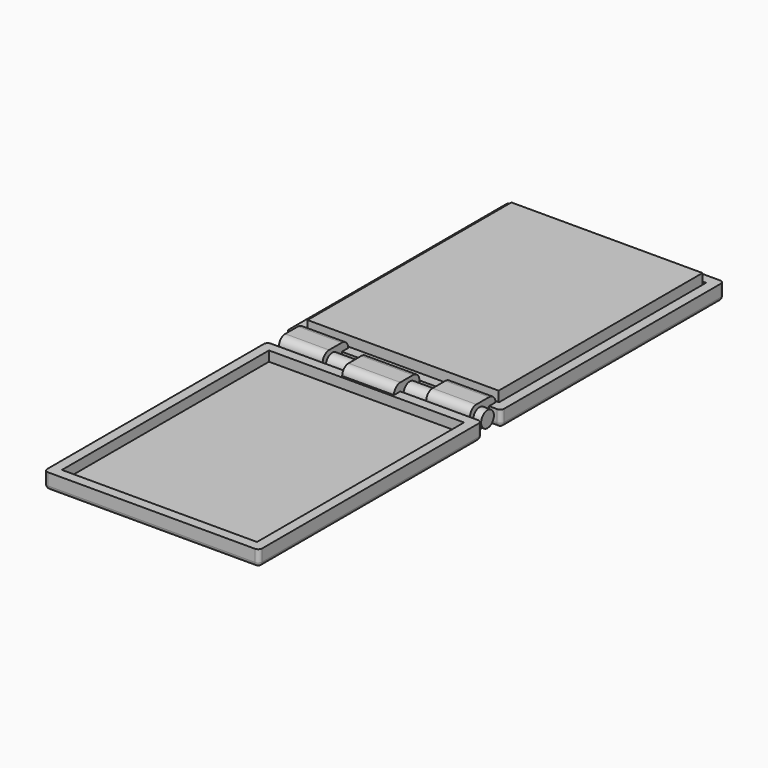
from build123d import *

# Parameters (mm, degrees)
F0_W      = 24
F0_H      = 32
F1_DEPTH  = 2.1
F3_W      = 27.0000016689
F3_H      = 35.0000016689
F3_W_2    = 24
F3_H_2    = 32
F4_DEPTH  = 4
F6_OFFSET = 0.25
F7_R      = 0.5
F5_W      = 35.0000016689
F5_H      = 2
F8_DEPTH  = 27.0000016689
F11_W     = 6.5
F11_H     = 2.9999983311
F11_H_2   = 1
F12_DEPTH = 3
F11_W_2   = 5.5000003338
F11_W_3   = 5.5000004172
F13_R     = 1
F14_DEPTH = 25
F15_R     = 1
F15_2_R   = 1
F15_3_R   = 1


with BuildPart() as f1:
    # F0 (on Top) → F1 (new body)
    with BuildSketch(Plane.XY):
        with Locations((12, 16)):
            Rectangle(F0_W, F0_H)
    extrude(amount=F1_DEPTH)


with BuildPart() as f4:
    # F3 (on offset) → F4 (new body)
    with BuildSketch(Plane.XY.offset(-1)):
        with Locations((12, 16)):
            Rectangle(F3_W, F3_H)
        with Locations((12, 16)):
            Rectangle(F3_W_2, F3_H_2, mode=Mode.SUBTRACT)
        with Locations((12, 16)):
            Rectangle(F3_W_2, F3_H_2)
    extrude(amount=F4_DEPTH)

    # F6: cut F1, made larger all round first
    f6_tool = offset(f1.part, amount=F6_OFFSET, kind=Kind.INTERSECTION, mode=Mode.PRIVATE)
    add(f6_tool, mode=Mode.SUBTRACT)

    # F7
    f7_edges = [f4.edges().sort_by_distance(p)[0] for p in [
        (-1.500001, -1.500001, 1),
        (25.500001, -1.500001, 1),
        (25.500001, 33.500001, 1),
        (-1.500001, 33.500001, 1),
        (-1.500001, 16, 3),
        (12, 33.500001, 3),
        (12, 33.500001, -1),
        (-1.500001, 16, -1),
        (25.500001, 16, 3),
        (25.500001, 16, -1),
        (12, -1.500001, 3),
        (12, -1.500001, -1),
    ]]
    fillet(f7_edges, radius=F7_R)

    # F5 (on face) → F8 (cut, through all)
    with BuildSketch(Plane.YZ.offset(25.5000008345)):
        with Locations((16, 2)):
            Rectangle(F5_W, F5_H)
    extrude(amount=-F8_DEPTH, mode=Mode.SUBTRACT)


with BuildPart() as f10_1:
    # F10: instance of F4
    add(f4.part.mirror(Plane.XZ.offset(3)))


with BuildPart() as f12:
    # F11 (on offset) → F12 (new body)
    with BuildSketch(Plane.XY.offset(-1)):
        with Locations((11.9999995828, -3)):
            Rectangle(F11_W, F11_H)
        with Locations((11.9999995828, -4.9999991655)):
            Rectangle(F11_W, F11_H_2)
    extrude(amount=F12_DEPTH)

    # F15
    f15_edges = [f12.edges().sort_by_distance(p)[0] for p in [
        (12, -5.499999, 2),
        (12, -1.500001, 2),
    ]]
    fillet(f15_edges, radius=F15_R)


with BuildPart() as f12b:
    # F11 (on offset) → F12, piece 2 (new body)
    with BuildSketch(Plane.XY.offset(-1)):
        with Locations((21.2500005841, -3)):
            Rectangle(F11_W_2, F11_H)
        with Locations((21.2500006258, -1.0000008345)):
            Rectangle(F11_W_3, F11_H_2)
    extrude(amount=F12_DEPTH)

    # F15#2
    f15_2_edges = [f12b.edges().sort_by_distance(p)[0] for p in [
        (21.250001, -0.500001, 2),
        (21.25, -4.499999, 2),
    ]]
    fillet(f15_2_edges, radius=F15_2_R)


with BuildPart() as f12c:
    # F11 (on offset) → F12, piece 3 (new body)
    with BuildSketch(Plane.XY.offset(-1)):
        with Locations((2.7499993742, -1.0000008345)):
            Rectangle(F11_W_3, F11_H_2)
        Polygon((5.4999995828, -1.5000008345), (-6.676e-07, -1.5000008345), (0, -4.4999991655), (5.4999995828, -4.4999991655), align=None)
    extrude(amount=F12_DEPTH)

    # F15#3
    f15_3_edges = [f12c.edges().sort_by_distance(p)[0] for p in [
        (2.749999, -0.500001, 2),
        (2.75, -4.499999, 2),
    ]]
    fillet(f15_3_edges, radius=F15_3_R)


with BuildPart() as f14:
    # F13 (on face) → F14 (new body)
    with BuildSketch(Plane(origin=(-9.179e-07, 0, 0), x_dir=(1.669e-07, -1, 0), z_dir=(-1, -1.669e-07, 0))):
        with Locations((3, 0.5)):
            Circle(F13_R)
    extrude(amount=-F14_DEPTH)


with BuildPart() as f16_1:
    # F16: copy of F4
    add(f4.part)


with BuildPart() as f17_1:
    # F17: copy of F4
    add(f4.part)


solid = Compound([f1.part, f4.part, f10_1.part, f12.part, f12b.part, f12c.part, f14.part, f16_1.part, f17_1.part])
